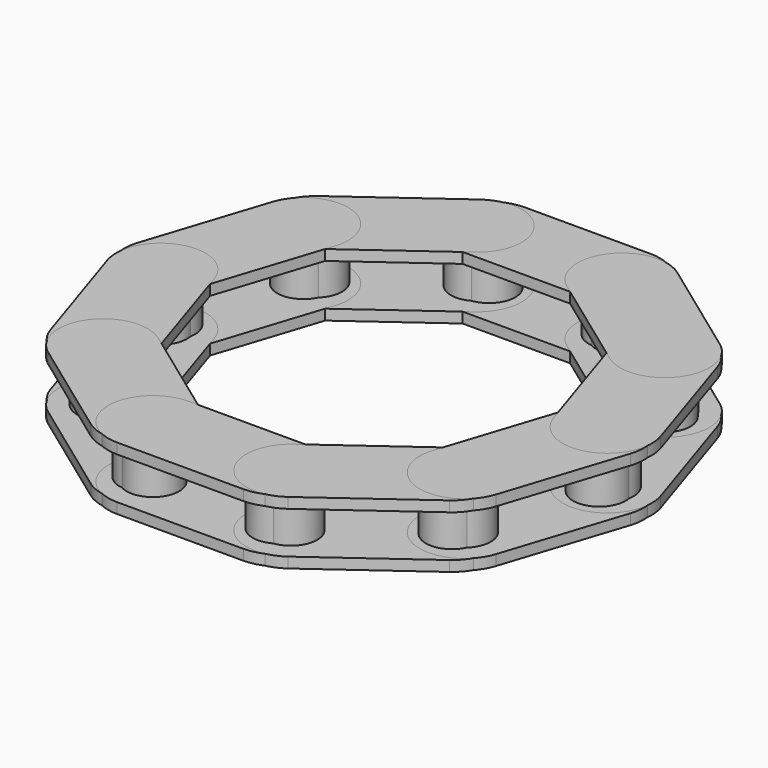
from build123d import *

# Parameters (mm, degrees)
F0_R     = 2.5
F1_DEPTH = 1
F2_DEPTH = 4
F3_R     = 2.5
F4_DEPTH = 1
F6_COUNT = 10


# Not quite as in the source:
# - a pattern or mirror of a feature is missing from the dataset's text; its kind, count and spacing are read off the source's solid
# - a feature names something its author has since deleted; it is built from what else it names


with BuildPart() as f1:
    # F0 (on Top) → F1 (new body)
    with BuildSketch(Plane.XY):
        with BuildLine():
            ThreePointArc((-6, 4.25), (-10.25, 0), (-6, -4.25))
            Line((-6, -4.25), (6, -4.25))
            ThreePointArc((6, -4.25), (10.25, 0), (6, 4.25))
            Line((6, 4.25), (-6, 4.25))
        make_face()
        with Locations((-6, 0)):
            Circle(F0_R, mode=Mode.SUBTRACT)
        with Locations((6, 0)):
            Circle(F0_R, mode=Mode.SUBTRACT)
        with Locations((-6, 0)):
            Circle(F0_R)
        with Locations((6, 0)):
            Circle(F0_R)
    extrude(amount=F1_DEPTH)


with BuildPart() as f1_copies_1:
    # F1_copies: instance of F1
    add(f1.part.mirror(Plane(origin=(0, 0, -2), x_dir=(-1, 0, 0), z_dir=(0, 0, -1))))


with BuildPart() as f1_1:
    add(f1.part)

    add(f1_copies_1.part)  # F2 merges F1_copies_1
    # F0 (on Top) → F2 (join)
    with BuildSketch(Plane.XY):
        with Locations((-6, 0)):
            Circle(F0_R)
        with Locations((6, 0)):
            Circle(F0_R)
    extrude(amount=-F2_DEPTH)

    # F3 (on face) → F4 (join)
    with BuildSketch(Plane(origin=(0, 0, -4), x_dir=(1, 0, 0), z_dir=(0, 0, -1))):
        with BuildLine():
            ThreePointArc((-6, 4.25), (-10.25, 0), (-6, -4.25))
            Line((-6, -4.25), (6, -4.25))
            ThreePointArc((6, -4.25), (10.25, 0), (6, 4.25))
            Line((6, 4.25), (-6, 4.25))
        make_face()
        with Locations((-6, 0)):
            Circle(F3_R, mode=Mode.SUBTRACT)
        with Locations((6, 0)):
            Circle(F3_R, mode=Mode.SUBTRACT)
    extrude(amount=F4_DEPTH)


with BuildPart() as f6_1:
    # F6: instance of F1
    add(f1_1.part.rotate(Axis((0, -20, 0), (0, 0, 1)), 1 * 360 / F6_COUNT))


with BuildPart() as f6_2:
    # F6: instance of F1
    add(f1_1.part.rotate(Axis((0, -20, 0), (0, 0, 1)), 2 * 360 / F6_COUNT))


with BuildPart() as f6_3:
    # F6: instance of F1
    add(f1_1.part.rotate(Axis((0, -20, 0), (0, 0, 1)), 3 * 360 / F6_COUNT))


with BuildPart() as f6_4:
    # F6: instance of F1
    add(f1_1.part.rotate(Axis((0, -20, 0), (0, 0, 1)), 4 * 360 / F6_COUNT))


with BuildPart() as f6_5:
    # F6: instance of F1
    add(f1_1.part.rotate(Axis((0, -20, 0), (0, 0, 1)), 5 * 360 / F6_COUNT))


with BuildPart() as f6_6:
    # F6: instance of F1
    add(f1_1.part.rotate(Axis((0, -20, 0), (0, 0, 1)), 6 * 360 / F6_COUNT))


with BuildPart() as f6_7:
    # F6: instance of F1
    add(f1_1.part.rotate(Axis((0, -20, 0), (0, 0, 1)), 7 * 360 / F6_COUNT))


with BuildPart() as f6_8:
    # F6: instance of F1
    add(f1_1.part.rotate(Axis((0, -20, 0), (0, 0, 1)), 8 * 360 / F6_COUNT))


with BuildPart() as f6_9:
    # F6: instance of F1
    add(f1_1.part.rotate(Axis((0, -20, 0), (0, 0, 1)), 9 * 360 / F6_COUNT))


solid = Compound([f1_1.part, f6_1.part, f6_2.part, f6_3.part, f6_4.part, f6_5.part, f6_6.part, f6_7.part, f6_8.part, f6_9.part])
